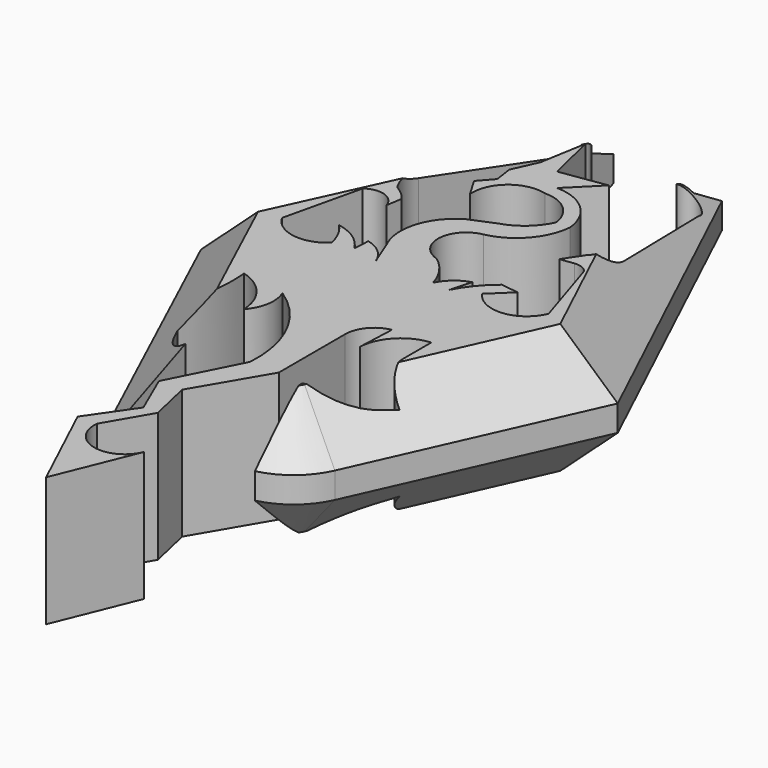
from build123d import *

# Parameters (mm, degrees)
F1_DEPTH     = 12.7
F2_T1_DEPTH  = 61.4894192219
F2_T3_DEPTH  = 60.6595144669
F2_T5_DEPTH  = 37.4346345762
F2_T10_DEPTH = 60.8311166964
F2_T15_ANGLE = 160.5521212616
F2_T20_DEPTH = 60.8311166964
F2_T25_ANGLE = 160.5521212616


# Not quite as in the source:
# - a fillet or chamfer that OpenCascade refuses, or shapes differently, is made with other operations: its cross-section is extruded or revolved along the edge and cut away or added


with BuildPart() as f1:
    # F0 (on Top) → F1 (new body)
    with BuildSketch(Plane.XY):
        with BuildLine():
            Line((38.2788181305, 17.8758297116), (42.2920919955, 24.7220024467))
            Line((42.2920919955, 24.7220024467), (42.2820188105, 32.8584946692))
            ThreePointArc((42.2820188105, 32.8584946692), (42.9440997072, 34.690736549), (44.6269139647, 35.6723666191))
            Line((44.6269139647, 35.6723666191), (44.4705858827, 31.9205336273))
            ThreePointArc((44.4705858827, 31.9205336273), (45.6310728705, 34.6386150419), (48.3005791903, 35.9068550169))
            Line((48.3005791903, 35.9068550169), (48.3005791903, 32.4676781893))
            ThreePointArc((48.3005791903, 32.4676781893), (48.8348924642, 30.7225209157), (50.2546578646, 29.5756421983))
            Line((50.2546578646, 29.5756421983), (49.394864589, 28.2468684018))
            ThreePointArc((49.394864589, 28.2468684018), (47.3924953639, 25.9852736124), (44.8100380599, 24.4183633476))
            Line((44.8100380599, 24.4183633476), (44.98494789, 18.4131488204))
            ThreePointArc((44.98494789, 18.4131488204), (47.8016399203, 19.8157230834), (49.7074984014, 22.3194546998))
            Line((49.7074984014, 22.3194546998), (59.6794784069, 44.5563644171))
            Line((59.6794784069, 44.5563644171), (44.9269972742, 75.77765733))
            Line((44.9269972742, 75.77765733), (44.417835772, 72.9466155171))
            ThreePointArc((44.417835772, 72.9466155171), (43.8763497816, 72.371486937), (43.8214614987, 71.5834721923))
            ThreePointArc((43.8214614987, 71.5834721923), (44.9290145189, 72.6595413512), (46.036567539, 71.5834721923))
            Line((46.036567539, 71.5834721923), (49.4444258511, 58.1224299967))
            ThreePointArc((49.4444258511, 58.1224299967), (49.4311906391, 56.2537383436), (48.5072657466, 54.6293780208))
            Line((48.5072657466, 54.6293780208), (47.3145134747, 52.8402514756))
            Line((47.3145134747, 52.8402514756), (48.6776567996, 53.0106425285))
            ThreePointArc((48.6776567996, 53.0106425285), (49.4221984033, 52.9229745419), (50.0408001244, 52.4994656444))
            Line((50.0408001244, 52.4994656444), (52.3411072791, 45.2577620745))
            ThreePointArc((52.3411072791, 45.2577620745), (49.496534757, 43.1348395296), (46.2921559811, 44.6613878012))
            Line((46.2921559811, 44.6613878012), (48.2516773045, 46.5357117355))
            Line((48.2516773045, 46.5357117355), (46.5477481484, 46.7913001776))
            ThreePointArc((46.5477481484, 46.7913001776), (45.0495064909, 45.3175304922), (43.9066551626, 43.5538366437))
            Line((43.9066551626, 43.5538366437), (44.5030331612, 45.6837452948))
            ThreePointArc((44.5030331612, 45.6837452948), (43.1415749719, 44.952040155), (42.2027260065, 43.7242276967))
            ThreePointArc((42.2027260065, 43.7242276967), (41.3363207449, 45.5819979858), (39.9024225771, 47.0468886197))
            ThreePointArc((39.9024225771, 47.0468886197), (37.9368947907, 49.8661923797), (40.2432084084, 52.4142682552))
            ThreePointArc((40.2432084084, 52.4142682552), (43.2781651475, 54.2049845256), (44.6734242141, 57.4408583343))
            ThreePointArc((44.6734242141, 57.4408583343), (43.1144375969, 60.6332712401), (39.817225188, 61.9562715292))
            Line((39.817225188, 61.9562715292), (42.6287092268, 64.767755568))
            Line((42.6287092268, 64.767755568), (38.113296032, 64.0861839056))
            Line((38.113296032, 64.0861839056), (36.9205437601, 69.0275803208))
            Line((36.9205437601, 69.0275803208), (36.1537747085, 64.5121708512))
            Line((36.1537747085, 64.5121708512), (35.046223551, 62.0414689183))
            Line((35.046223551, 62.0414689183), (35.3018119931, 60.2523423731))
            Line((35.3018119931, 60.2523423731), (34.1090597212, 58.8891990483))
            Line((34.1090597212, 58.8891990483), (35.216614604, 57.0148788393))
            ThreePointArc((35.216614604, 57.0148788393), (36.4787140011, 59.9990779117), (39.6468304098, 60.6783255935))
            ThreePointArc((39.6468304098, 60.6783255935), (42.100861171, 59.7637799228), (43.3102808893, 57.4408583343))
            ThreePointArc((43.3102808893, 57.4408583343), (41.960859951, 55.6347382447), (39.987616241, 54.5441806316))
            Line((39.987616241, 54.5441806316), (37.5169217587, 53.521823138))
            ThreePointArc((37.5169217587, 53.521823138), (35.2577529504, 50.8211890197), (35.1314172149, 47.302480787))
            Line((35.1314172149, 47.302480787), (36.494564265, 43.8946224749))
            ThreePointArc((36.494564265, 43.8946224749), (35.5191674638, 45.2611219807), (34.0238660574, 46.024531126))
            Line((34.0238660574, 46.024531126), (33.9386686683, 44.4057993591))
            ThreePointArc((33.9386686683, 44.4057993591), (32.5250680188, 45.9137846149), (30.6160058826, 46.7061027884))
            ThreePointArc((30.6160058826, 46.7061027884), (31.4840333326, 45.4817930881), (31.9791510701, 44.0650135279))
            ThreePointArc((31.9791510701, 44.0650135279), (29.0027298162, 43.1420138964), (26.4413785189, 44.9169762433))
            Line((26.4413785189, 44.9169762433), (28.2305050641, 52.5846593082))
            ThreePointArc((28.2305050641, 52.5846593082), (30.0752112346, 52.9015778311), (31.3827730715, 51.5623018146))
            Line((31.3827730715, 51.5623018146), (31.6383615136, 53.0958399177))
            ThreePointArc((31.6383615136, 53.0958399177), (30.9888271445, 53.8193992901), (30.1900226623, 54.3737858534))
            ThreePointArc((30.1900226623, 54.3737858534), (29.5328449453, 55.9706841256), (29.593648389, 57.6964505017))
            Line((29.593648389, 57.6964505017), (32.9163111746, 70.8167105913))
            ThreePointArc((32.9163111746, 70.8167105913), (33.7093855935, 71.7795807909), (34.7906313837, 71.1574926972))
            ThreePointArc((34.7906313837, 71.1574926972), (34.7651749092, 72.4631986698), (33.5519872606, 72.9466155171))
            Line((33.5519872606, 72.9466155171), (33.5519872606, 76.6831859946))
            Line((33.5519872606, 76.6831859946), (18.7778156251, 44.5563644171))
            Line((18.7778156251, 44.5563644171), (33.3570353687, 13.0645893514))
            Line((33.3570353687, 13.0645893514), (33.3570353687, 24.4183633476))
            ThreePointArc((33.3570353687, 24.4183633476), (30.754145435, 26.167413579), (29.0718954057, 28.8139674813))
            ThreePointArc((29.0718954057, 28.8139674813), (29.8771193905, 32.3095735456), (29.9375038594, 35.8962155879))
            ThreePointArc((29.9375038594, 35.8962155879), (32.545088234, 34.1789060872), (33.6360111833, 31.2534086406))
            ThreePointArc((33.6360111833, 31.2534086406), (34.5240159071, 33.128980926), (34.2655442655, 35.1879894733))
            ThreePointArc((34.2655442655, 35.1879894733), (38.2849845666, 30.6609560826), (39.4591912627, 24.7220024467))
            Line((39.4591912627, 24.7220024467), (35.996761173, 17.8758297116))
            Line((35.996761173, 17.8758297116), (37.8066673875, 13.705172576))
            Line((37.8066673875, 13.705172576), (34.8163843155, 9.3771321699))
            Line((34.8163843155, 9.3771321699), (39.2231196165, 0))
            Line((39.2231196165, 0), (42.4494743347, 7.9606827348))
            ThreePointArc((42.4494743347, 7.9606827348), (38.9638620653, 6.181357436), (36.7049872875, 9.3771321699))
            Line((36.7049872875, 9.3771321699), (39.2231196165, 13.705172576))
            Line((39.2231196165, 13.705172576), (38.2788181305, 17.8758297116))
        make_face()
    extrude(amount=F1_DEPTH)

    # F2: chamfer of 5.08 on 10 edges, made by hand

    # F2_s2 → F2_t1 (cut)
    with BuildSketch(Plane(origin=(40.423720467, 87.9024345312, 0), x_dir=(0, 0, 1), z_dir=(-0.4178083615, -0.9085351799, 0))):
        Polygon((7.62, 1.5557155161), (12.7, -3.5242844839), (12.7, 1.5557155161), align=None)
        Polygon((5.08, 1.5557155161), (0, -3.5242844839), (0, 1.5557155161), align=None)
    extrude(amount=F2_T1_DEPTH, mode=Mode.SUBTRACT)

    # F2_s4 → F2_t3 (cut)
    with BuildSketch(Plane(origin=(-0.736952526, 1.5596434572, 0), x_dir=(0, 0, 1), z_dir=(-0.4272216023, 0.9041469474, 0))):
        Polygon((7.62, 72.9944596236), (12.7, 67.9144596236), (12.7, 72.9944596236), align=None)
        Polygon((5.08, 72.9944596236), (0, 67.9144596236), (0, 72.9944596236), align=None)
    extrude(amount=F2_T3_DEPTH, mode=Mode.SUBTRACT)

    # F2_s6 → F2_t5 (cut)
    with BuildSketch(Plane(origin=(16.6557348467, 37.141277044, 0), x_dir=(0, 0, 1), z_dir=(0.4091826653, 0.91245249, 0))):
        Polygon((7.62, 36.2229967242), (12.7, 31.1429967242), (12.7, 36.2229967242), align=None)
        Polygon((5.08, 36.2229967242), (0, 31.1429967242), (0, 36.2229967242), align=None)
    extrude(amount=F2_T5_DEPTH, mode=Mode.SUBTRACT)


with BuildPart() as f2_tool8:
    # F2_s9 → F2_t10 (new body)
    with BuildSketch(Plane(origin=(-19.1610255807, 41.3886832236, 0), x_dir=(0, 0, 1), z_dir=(0.4201163127, -0.9074702661, 0))):
        Polygon((7.62, -35.7591648667), (12.7, -40.8391648667), (12.7, -35.7591648667), align=None)
    extrude(amount=F2_T10_DEPTH)

    split(bisect_by=Plane(origin=(21.465639244, -10.8561787862, 0), x_dir=(0, 0, 1), z_dir=(-0.8923664741, 0.4513115065, 0)), keep=Keep.TOP)


with BuildPart() as f1_1:
    add(f1.part)

    # F2_t7: cut F2_tool8
    add(f2_tool8.part, mode=Mode.SUBTRACT)


with BuildPart() as f2_tool13:
    # F2_s14 → F2_t15 (revolve)
    with BuildSketch(Plane(origin=(2.3486048787, 28.532346778, 0), x_dir=(0, 0, 1), z_dir=(0.0820363131, 0.996629341, 0))):
        Polygon((7.62, 34.2474692794), (12.7, 39.3274692794), (12.7, 34.2474692794), align=None)
    revolve(axis=Axis((43.3856729768, 25.154431211, 12.7), (0, 0, 1)), revolution_arc=F2_T15_ANGLE)

    split(bisect_by=Plane(origin=(45.4826703508, 1.3247430391, 0), x_dir=(0, 0, 1), z_dir=(0.9995760983, 0.0291139783, 0)), keep=Keep.TOP)


with BuildPart() as f1_2:
    add(f1_1.part)

    # F2_t12: cut F2_tool13
    add(f2_tool13.part, mode=Mode.SUBTRACT)


with BuildPart() as f2_tool18:
    # F2_s19 → F2_t20 (new body)
    with BuildSketch(Plane(origin=(-19.1610255807, 41.3886832236, 0), x_dir=(0, 0, 1), z_dir=(0.4201163127, -0.9074702661, 0))):
        Polygon((5.08, -35.7591648667), (0, -40.8391648667), (0, -35.7591648667), align=None)
    extrude(amount=F2_T20_DEPTH)

    split(bisect_by=Plane(origin=(21.465639244, -10.8561787862, 0), x_dir=(0, 0, 1), z_dir=(-0.8923664741, 0.4513115065, 0)), keep=Keep.TOP)


with BuildPart() as f1_3:
    add(f1_2.part)

    # F2_t17: cut F2_tool18
    add(f2_tool18.part, mode=Mode.SUBTRACT)


with BuildPart() as f2_tool23:
    # F2_s24 → F2_t25 (revolve)
    with BuildSketch(Plane(origin=(2.3486048787, 28.532346778, 0), x_dir=(0, 0, 1), z_dir=(0.0820363131, 0.996629341, 0))):
        Polygon((5.08, 34.2474692794), (0, 39.3274692794), (0, 34.2474692794), align=None)
    revolve(axis=Axis((43.3856729768, 25.154431211, 0), (0, 0, 1)), revolution_arc=F2_T25_ANGLE)

    split(bisect_by=Plane(origin=(45.4826703508, 1.3247430391, 0), x_dir=(0, 0, 1), z_dir=(0.9995760983, 0.0291139783, 0)), keep=Keep.TOP)


with BuildPart() as f1_4:
    add(f1_3.part)

    # F2_t22: cut F2_tool23
    add(f2_tool23.part, mode=Mode.SUBTRACT)


solid = f1_4.part
